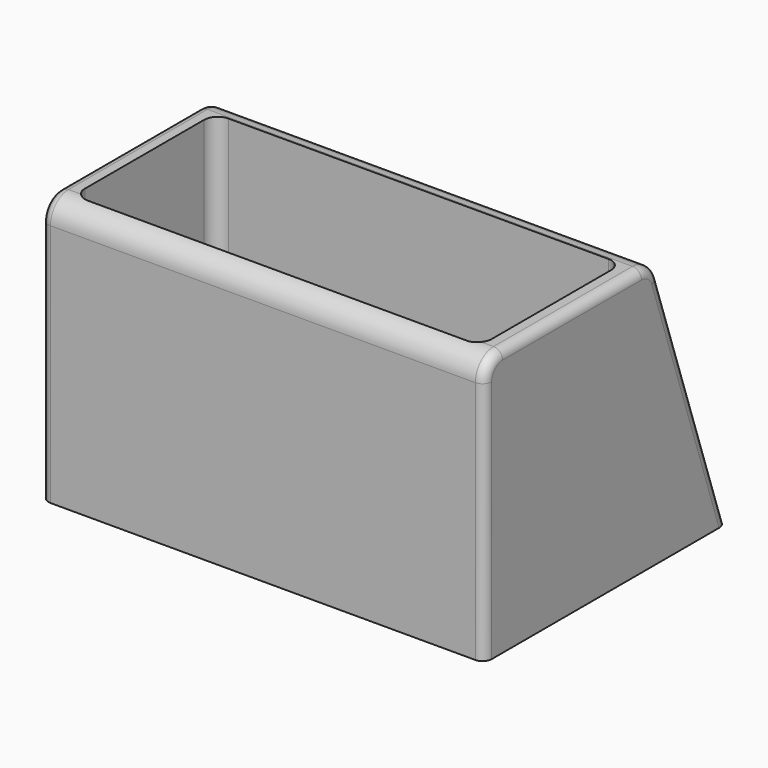
from build123d import *

# Parameters (mm, degrees)
F1_DEPTH    = 98
F3_DEPTH    = 39
F4_T1_DEPTH = 123
F4_T3_DEPTH = 115.9227425884
F5_R        = 2


# Not quite as in the source:
# - a fillet or chamfer that OpenCascade refuses, or shapes differently, is made with other operations: its cross-section is extruded or revolved along the edge and cut away or added


with BuildPart() as f1:
    # F0 (on Right) → F1 (new body)
    with BuildSketch(Plane.YZ):
        Polygon((0, 59), (0, 0), (67, 0), (47, 59), align=None)
    extrude(amount=F1_DEPTH)

    # F2 (on face) → F3 (cut)
    with BuildSketch(Plane.XY.offset(59)):
        with BuildLine():
            Line((91, 43), (7, 43))
            ThreePointArc((7, 43), (4.8786796564, 42.1213203436), (4, 40))
            Line((4, 40), (4, 7))
            ThreePointArc((4, 7), (4.8786796564, 4.8786796564), (7, 4))
            Line((7, 4), (91, 4))
            ThreePointArc((91, 4), (93.1213203436, 4.8786796564), (94, 7))
            Line((94, 7), (94, 40))
            ThreePointArc((94, 40), (93.1213203436, 42.1213203436), (91, 43))
        make_face()
    extrude(amount=-F3_DEPTH, mode=Mode.SUBTRACT)

    # F4: fillet of radius 5 on 2 edges, made by hand

    # F4_s2 → F4_t1 (cut)
    with BuildSketch(Plane.YZ.offset(-12.5)):
        with BuildLine():
            ThreePointArc((0, 54), (1.4644660941, 57.5355339059), (5, 59))
            Line((5, 59), (0, 59))
            Line((0, 59), (0, 54))
        make_face()
    extrude(amount=F4_T1_DEPTH, mode=Mode.SUBTRACT)

    # F4_s4 → F4_t3 (cut)
    with BuildSketch(Plane.YZ.offset(-8.9613712942)):
        with BuildLine():
            ThreePointArc((43.4154514823, 59), (46.3286986372, 58.063617971), (48.1507808794, 55.6051964058))
            Line((48.1507808794, 55.6051964058), (47, 59))
            Line((47, 59), (43.4154514823, 59))
        make_face()
    extrude(amount=F4_T3_DEPTH, mode=Mode.SUBTRACT)

    # F5
    f5_edges = [f1.edges().sort_by_distance(p)[0] for p in [
        (0, 24.207726, 59),
        (98, 24.207726, 59),
        (0, 0, 27),
        (98, 0, 27),
        (0, 1.464466, 57.535534),
        (0, 46.328699, 58.063618),
        (0, 57.57539, 27.802598),
        (98, 1.464466, 57.535534),
        (98, 46.328699, 58.063618),
        (98, 57.57539, 27.802598),
    ]]
    fillet(f5_edges, radius=F5_R)


solid = f1.part
